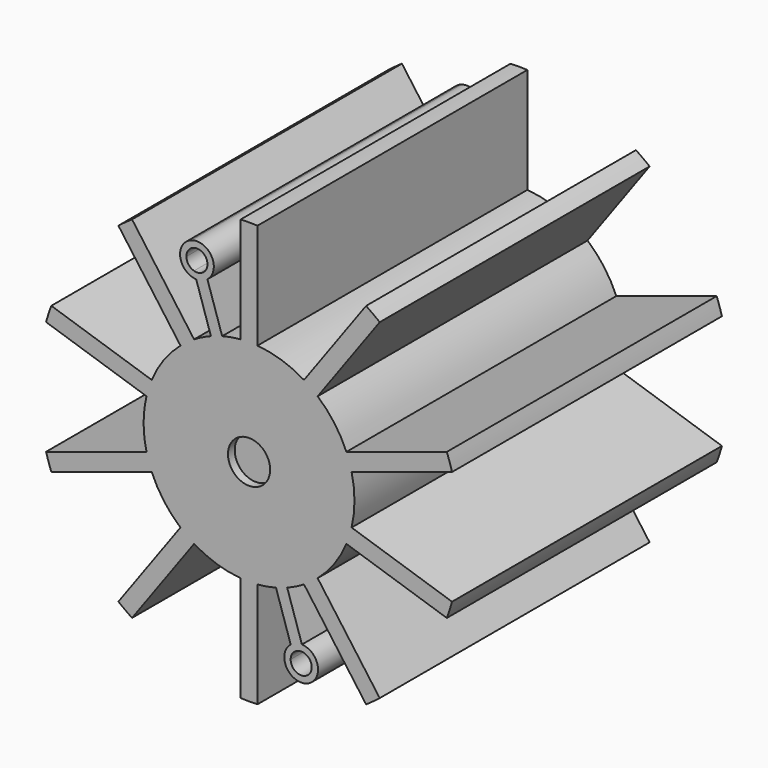
from build123d import *

# Parameters (mm, degrees)
F0_R      = 25
F1_DEPTH  = 40
F2_R      = 2.5
F3_DEPTH  = 1
F5_DEPTH  = 40.001
F7_DEPTH  = 40
F8_R      = 2.5
F9_DEPTH  = 1
F10_R     = 1.5
F11_DEPTH = 5


with BuildPart() as f1:
    # F0 (on Front) → F1 (new body)
    with BuildSketch(Plane.XZ):
        Circle(F0_R)
    extrude(amount=F1_DEPTH)

    # F2 (on face) → F3 (cut)
    with BuildSketch(Plane(origin=(0, 0, 0), x_dir=(-1, 0, 0), z_dir=(0, 1, 0))):
        Circle(F2_R)
    extrude(amount=-F3_DEPTH, mode=Mode.SUBTRACT)

    # F4 (on face) → F5 (cut, through all)
    with BuildSketch(Plane(origin=(0, 0, 0), x_dir=(-1, 0, 0), z_dir=(0, 1, 0))):
        with BuildLine():
            ThreePointArc((8.1327834988, 9.4925145542), (10.1127124297, 7.3473156537), (11.5410861355, 4.8013884256))
            Line((11.5410861355, 4.8013884256), (23.4483671681, 8.6702985617))
            ThreePointArc((23.4483671681, 8.6702985617), (20.2254248594, 14.6946313073), (15.4918878906, 19.6214527899))
            Line((15.4918878906, 19.6214527899), (8.1327834988, 9.4925145542))
        make_face()
        with BuildLine():
            ThreePointArc((1, 12.4599357944), (3.8627124297, 11.8882064537), (6.5147495101, 10.6680850588))
            Line((6.5147495101, 10.6680850588), (13.8738539018, 20.7970232945))
            ThreePointArc((13.8738539018, 20.7970232945), (7.7254248594, 23.7764129074), (1, 24.9799919936))
            Line((1, 24.9799919936), (1, 12.4599357944))
        make_face()
        with BuildLine():
            ThreePointArc((-6.5147495101, 10.6680850588), (-3.8627124297, 11.8882064537), (-1, 12.4599357944))
            Line((-1, 12.4599357944), (-1, 24.9799919936))
            ThreePointArc((-1, 24.9799919936), (-7.7254248594, 23.7764129074), (-13.8738539018, 20.7970232945))
            Line((-13.8738539018, 20.7970232945), (-6.5147495101, 10.6680850588))
        make_face()
        with BuildLine():
            ThreePointArc((-11.5410861355, 4.8013884256), (-10.1127124297, 7.3473156537), (-8.1327834988, 9.4925145542))
            Line((-8.1327834988, 9.4925145542), (-15.4918878906, 19.6214527899))
            ThreePointArc((-15.4918878906, 19.6214527899), (-20.2254248594, 14.6946313073), (-23.4483671681, 8.6702985617))
            Line((-23.4483671681, 8.6702985617), (-11.5410861355, 4.8013884256))
        make_face()
        with BuildLine():
            ThreePointArc((-12.1591201242, -2.899275393), (-12.5, 0), (-12.1591201242, 2.899275393))
            Line((-12.1591201242, 2.899275393), (-24.0664011569, 6.7681855291))
            ThreePointArc((-24.0664011569, 6.7681855291), (-25, 0), (-24.0664011569, -6.7681855291))
            Line((-24.0664011569, -6.7681855291), (-12.1591201242, -2.899275393))
        make_face()
        with BuildLine():
            Line((-15.4918878906, -19.6214527899), (-8.1327834988, -9.4925145542))
            ThreePointArc((-8.1327834988, -9.4925145542), (-10.1127124297, -7.3473156537), (-11.5410861355, -4.8013884256))
            Line((-11.5410861355, -4.8013884256), (-23.4483671681, -8.6702985617))
            ThreePointArc((-23.4483671681, -8.6702985617), (-20.2254248594, -14.6946313073), (-15.4918878906, -19.6214527899))
        make_face()
        with BuildLine():
            Line((-1, -24.9799919936), (-1, -12.4599357944))
            ThreePointArc((-1, -12.4599357944), (-3.8627124297, -11.8882064537), (-6.5147495101, -10.6680850588))
            Line((-6.5147495101, -10.6680850588), (-13.8738539018, -20.7970232945))
            ThreePointArc((-13.8738539018, -20.7970232945), (-7.7254248594, -23.7764129074), (-1, -24.9799919936))
        make_face()
        with BuildLine():
            Line((13.8738539018, -20.7970232945), (6.5147495101, -10.6680850588))
            ThreePointArc((6.5147495101, -10.6680850588), (3.8627124297, -11.8882064537), (1, -12.4599357944))
            Line((1, -12.4599357944), (1, -24.9799919936))
            ThreePointArc((1, -24.9799919936), (7.7254248594, -23.7764129074), (13.8738539018, -20.7970232945))
        make_face()
        with BuildLine():
            Line((23.4483671681, -8.6702985617), (11.5410861355, -4.8013884256))
            ThreePointArc((11.5410861355, -4.8013884256), (10.1127124297, -7.3473156537), (8.1327834988, -9.4925145542))
            Line((8.1327834988, -9.4925145542), (15.4918878906, -19.6214527899))
            ThreePointArc((15.4918878906, -19.6214527899), (20.2254248594, -14.6946313073), (23.4483671681, -8.6702985617))
        make_face()
        with BuildLine():
            ThreePointArc((12.1591201242, 2.899275393), (12.4144875358, 1.4596229731), (12.5, 0))
            ThreePointArc((12.5, 0), (12.4144875358, -1.4596229731), (12.1591201242, -2.899275393))
            Line((12.1591201242, -2.899275393), (24.0664011569, -6.7681855291))
            ThreePointArc((24.0664011569, -6.7681855291), (24.7655004888, -3.4161360539), (25, 0))
            ThreePointArc((25, 0), (24.7655004888, 3.4161360539), (24.0664011569, 6.7681855291))
            Line((24.0664011569, 6.7681855291), (12.1591201242, 2.899275393))
        make_face()
    extrude(amount=-F5_DEPTH, mode=Mode.SUBTRACT)

    # F6 (on face) → F7 (join)
    with BuildSketch(Plane(origin=(0, 0, 0), x_dir=(-1, 0, 0), z_dir=(0, 1, 0))):
        with BuildLine():
            ThreePointArc((2.5, 0), (2.0225424859, 1.4694631307), (0.7725424859, 2.3776412907))
            ThreePointArc((0.7725424859, 2.3776412907), (-2.0225424859, -1.4694631307), (2.5, 0))
        make_face()
        with BuildLine():
            ThreePointArc((-3.1909113793, -12.0858630048), (-3.8627124297, -11.8882064537), (-4.5223905021, -11.6532392126))
            Line((-4.5223905021, -11.6532392126), (-6.2671362955, -17.0230146177))
            ThreePointArc((-6.2671362955, -17.0230146177), (-5.5623058987, -17.1190172933), (-4.9356571727, -17.4556384098))
            Line((-4.9356571727, -17.4556384098), (-3.1909113793, -12.0858630048))
        make_face()
        with BuildLine():
            Line((-6.5260565798, -17.819889314), (-6.2671362955, -17.0230146177))
            ThreePointArc((-6.2671362955, -17.0230146177), (-7.5635259169, -20.465705145), (-4.1803398875, -19.0211303259))
            ThreePointArc((-4.1803398875, -19.0211303259), (-4.379039603, -18.1520404081), (-4.9356571727, -17.4556384098))
            Line((-4.9356571727, -17.4556384098), (-5.194577457, -18.2525131061))
            ThreePointArc((-5.194577457, -18.2525131061), (-4.9982436481, -18.6147456794), (-4.9303398875, -19.0211303259))
            ThreePointArc((-4.9303398875, -19.0211303259), (-6.9321224806, -20.0197908952), (-6.5260565798, -17.819889314))
        make_face()
        with BuildLine():
            ThreePointArc((3.1909113793, 12.0858630048), (3.5281963151, 11.9917401057), (3.8627124297, 11.8882064537))
            Line((3.8627124297, 11.8882064537), (5.5623058987, 17.1190172933))
            ThreePointArc((5.5623058987, 17.1190172933), (5.233895582, 17.2592440706), (4.9356571727, 17.4556384098))
            Line((4.9356571727, 17.4556384098), (3.1909113793, 12.0858630048))
        make_face()
        with BuildLine():
            Line((5.5623058987, 17.1190172933), (3.8627124297, 11.8882064537))
            ThreePointArc((3.8627124297, 11.8882064537), (4.1941972051, 11.7753432988), (4.5223905021, 11.6532392126))
            Line((4.5223905021, 11.6532392126), (6.2671362955, 17.0230146177))
            ThreePointArc((6.2671362955, 17.0230146177), (5.9104186578, 17.0394283983), (5.5623058987, 17.1190172933))
        make_face()
        with BuildLine():
            ThreePointArc((6.7983738762, 20.9232433585), (4.4184536322, 19.9675746314), (4.9356571727, 17.4556384098))
            Line((4.9356571727, 17.4556384098), (5.194577457, 18.2525131061))
            ThreePointArc((5.194577457, 18.2525131061), (5.1567490659, 19.7385993706), (6.5666111305, 20.2099509713))
            Line((6.5666111305, 20.2099509713), (6.7983738762, 20.9232433585))
        make_face()
        with BuildLine():
            Line((6.5260565798, 17.819889314), (6.2671362955, 17.0230146177))
            ThreePointArc((6.2671362955, 17.0230146177), (7.6249147066, 17.6379442965), (8.1803398875, 19.0211303259))
            ThreePointArc((8.1803398875, 19.0211303259), (7.7983738762, 20.1967008305), (6.7983738762, 20.9232433585))
            Line((6.7983738762, 20.9232433585), (6.5666111305, 20.2099509713))
            ThreePointArc((6.5666111305, 20.2099509713), (7.1916111305, 19.7558618913), (7.4303398875, 19.0211303259))
            ThreePointArc((7.4303398875, 19.0211303259), (7.1790004568, 18.2693477328), (6.5260565798, 17.819889314))
        make_face()
        with BuildLine():
            ThreePointArc((-4.9356571727, -17.4556384098), (-5.5623058987, -17.1190172933), (-6.2671362955, -17.0230146177))
            Line((-6.2671362955, -17.0230146177), (-6.5260565798, -17.819889314))
            ThreePointArc((-6.5260565798, -17.819889314), (-5.7940686445, -17.8323096805), (-5.194577457, -18.2525131061))
            Line((-5.194577457, -18.2525131061), (-4.9356571727, -17.4556384098))
        make_face()
        with BuildLine():
            ThreePointArc((4.9356571727, 17.4556384098), (5.233895582, 17.2592440706), (5.5623058987, 17.1190172933))
            Line((5.5623058987, 17.1190172933), (5.7940686445, 17.8323096805))
            ThreePointArc((5.7940686445, 17.8323096805), (5.4628708429, 17.9975395043), (5.194577457, 18.2525131061))
            Line((5.194577457, 18.2525131061), (4.9356571727, 17.4556384098))
        make_face()
        with BuildLine():
            Line((5.7940686445, 17.8323096805), (5.5623058987, 17.1190172933))
            ThreePointArc((5.5623058987, 17.1190172933), (5.9104186578, 17.0394283983), (6.2671362955, 17.0230146177))
            Line((6.2671362955, 17.0230146177), (6.5260565798, 17.819889314))
            ThreePointArc((6.5260565798, 17.819889314), (6.1591329483, 17.7713102326), (5.7940686445, 17.8323096805))
        make_face()
    extrude(amount=-F7_DEPTH)

    # F8 (on face) → F9 (cut)
    with BuildSketch(Plane.XZ.offset(40)):
        Circle(F8_R)
    extrude(amount=-F9_DEPTH, mode=Mode.SUBTRACT)

    # F10 (on face) → F11 (cut)
    with BuildSketch(Plane(origin=(0, 0, 0), x_dir=(-1, 0, 0), z_dir=(0, 1, 0))):
        with Locations((10, 0)):
            Circle(F10_R)
        with Locations((-10, -0.6205414017)):
            Circle(F10_R)
        with Locations((0, -10)):
            Circle(F10_R)
        with Locations((0, 10)):
            Circle(F10_R)
    extrude(amount=-F11_DEPTH, mode=Mode.SUBTRACT)


solid = f1.part
